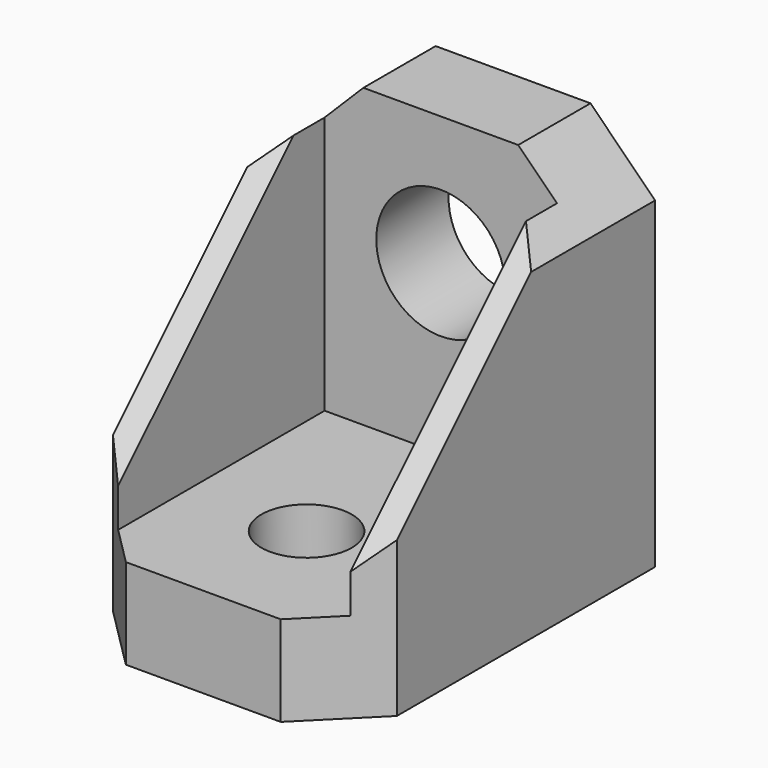
from build123d import *

# Parameters (mm, degrees)
F0_W        = 2
F0_H        = 23
F0_W_2      = 18
F0_R        = 3.5
F1_DEPTH    = 7
F2_DEPTH    = 23
F3_R        = 5
F4_DEPTH    = 25
F5_SIZE     = 23
F6_T1_DEPTH = 32.7168298797
F6_T3_DEPTH = 32.7168298797


# Not quite as in the source:
# - a fillet or chamfer that OpenCascade refuses, or shapes differently, is made with other operations: its cross-section is extruded or revolved along the edge and cut away or added


with BuildPart() as f1:
    # F0 (on Top) → F1 (new body)
    with BuildSketch(Plane.XY):
        with Locations((-10, -3.5)):
            Rectangle(F0_W, F0_H)
        with Locations((0, -3.5)):
            Rectangle(F0_W_2, F0_H)
        with Locations((0, -5)):
            Circle(F0_R, mode=Mode.SUBTRACT)
        with Locations((10, -3.5)):
            Rectangle(F0_W, F0_H)
        Polygon((9, 8), (11, 8), (11, 15), (-11, 15), (-11, 8), (-9, 8), align=None)
    extrude(amount=-F1_DEPTH)

    # F0 (on Top) → F2 (join)
    with BuildSketch(Plane.XY):
        Polygon((9, 8), (11, 8), (11, 15), (-11, 15), (-11, 8), (-9, 8), align=None)
        with Locations((-10, -3.5)):
            Rectangle(F0_W, F0_H)
        with Locations((10, -3.5)):
            Rectangle(F0_W, F0_H)
    extrude(amount=F2_DEPTH)

    # F3 (on face) → F4 (cut)
    with BuildSketch(Plane.XZ.offset(-8)):
        with Locations((0, 13)):
            Circle(F3_R)
    extrude(amount=-F4_DEPTH, mode=Mode.SUBTRACT)

    # F5
    f5_edges = [f1.edges().sort_by_distance(p)[0] for p in [
        (10, -15, 23),
        (-10, -15, 23),
    ]]
    chamfer(f5_edges, length=F5_SIZE)

    # F6: chamfer of 5 on 4 edges, made by hand

    # F6_s2 → F6_t1 (cut)
    with BuildSketch(Plane.XY.offset(-19.8584149398)):
        Polygon((-6, -15), (-11, -10), (-11, -15), align=None)
        Polygon((6, -15), (11, -10), (11, -15), align=None)
    extrude(amount=F6_T1_DEPTH, mode=Mode.SUBTRACT)

    # F6_s4 → F6_t3 (cut)
    with BuildSketch(Plane.XZ.offset(-27.8584149398)):
        Polygon((-11, 18), (-6, 23), (-11, 23), align=None)
        Polygon((11, 18), (6, 23), (11, 23), align=None)
    extrude(amount=F6_T3_DEPTH, mode=Mode.SUBTRACT)


solid = f1.part
